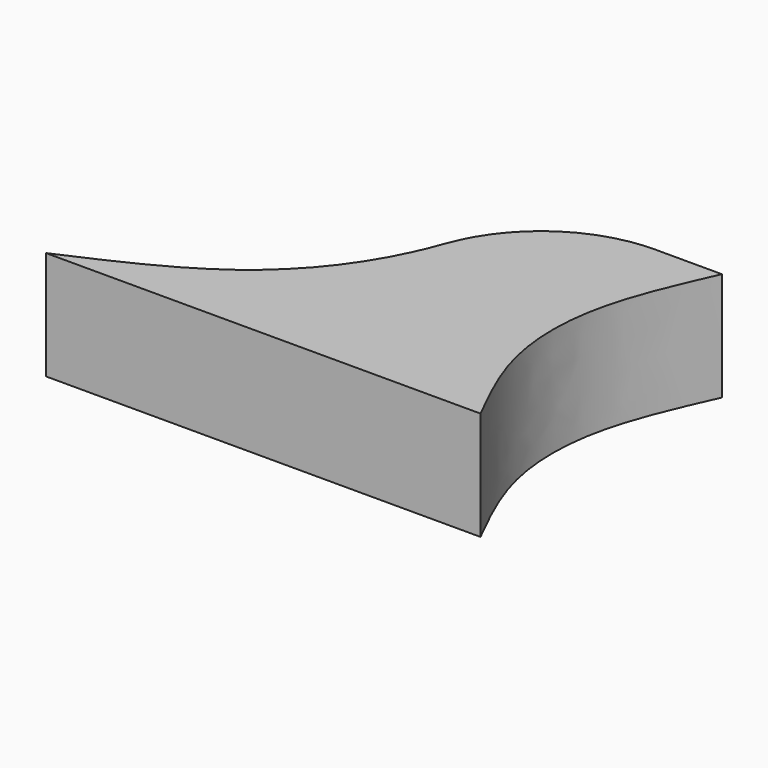
from build123d import *

# Parameters (mm, degrees)
F1_DEPTH = 25
F2_R     = 32.913540843


with BuildPart() as f1:
    # F0 (on Top) → F1 (new body)
    with BuildSketch(Plane.XY):
        with BuildLine():
            add(Edge.make_bspline(
                [(-39.2333641648, 0), (-27.7979598726, 5.0517939803), (-5.8928164583, 14.728782114), (13.7537860075, 40.0800253408), (18.095766656, 59.7227230679), (20.2540475875, 69.486575876)],
                knots=[0, 0, 0, 0, 0.354553063, 0.6791658164, 1, 1, 1, 1], degree=3))
            Line((-39.2333641648, 0), (60.7666358352, 0))
            add(Edge.make_bspline(
                [(60.7666358352, 0), (57.2575599986, 6.9981081509), (50.237319798, 20.9984895783), (49.931864791, 45.321172526), (57.0784932504, 61.2607026379), (60.7666358352, 69.486575876)],
                knots=[0, 0, 0, 0, 0.3259841606, 0.65216234, 1, 1, 1, 1], degree=3))
            Line((60.7666358352, 69.486575876), (52.7530318439, 69.486575876))
            Line((52.7530318439, 69.486575876), (20.2540475875, 69.486575876))
        make_face()
    extrude(amount=F1_DEPTH)

    # F2
    f2_edges = [f1.edges().sort_by_distance(p)[0] for p in [
        (20.254048, 69.486576, 12.5),
    ]]
    fillet(f2_edges, radius=F2_R)


solid = f1.part
